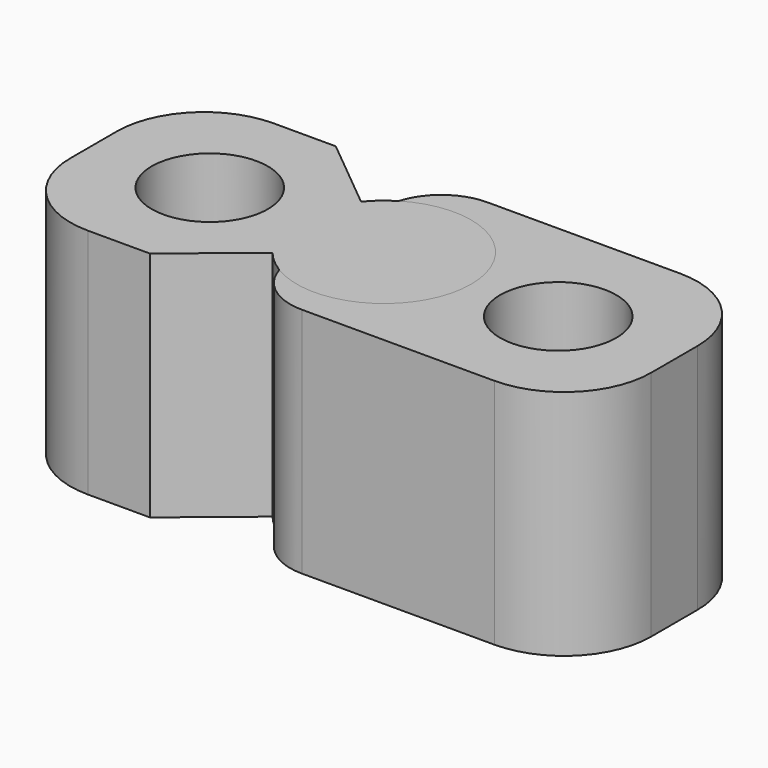
from build123d import *

# Parameters (mm, degrees)
F1_DEPTH    = 4
F2_DEPTH    = 4
F3_R        = 1.5
F3_2_R      = 1.5
F4_T1_DEPTH = 13.1378583471
F5_D        = 2
F5_2_D      = 2


# Not quite as in the source:
# - a fillet or chamfer that OpenCascade refuses, or shapes differently, is made with other operations: its cross-section is extruded or revolved along the edge and cut away or added


with BuildPart() as f1:
    # F0 (on Top) → F1 (new body)
    with BuildSketch(Plane.XY):
        with BuildLine():
            Line((-1.1581599978, 0.9532394345), (-2.4299456272, 2))
            Line((-2.4299456272, 2), (-5, 2))
            Line((-5, 2), (-5, -2))
            Line((-5, -2), (-2.4299456272, -2))
            Line((-2.4299456272, -2), (-1.1581599978, -0.9532394345))
            ThreePointArc((-1.1581599978, -0.9532394345), (-1.5, 0), (-1.1581599978, 0.9532394345))
        make_face()
        with BuildLine():
            ThreePointArc((1.5, 0), (0.7378123545, 1.3059988245), (-0.7741772393, 1.2847760902))
            ThreePointArc((-0.7741772393, 1.2847760902), (-0.9802861511, 1.135358561), (-1.1581599978, 0.9532394345))
            ThreePointArc((-1.1581599978, 0.9532394345), (-1.5, 0), (-1.1581599978, -0.9532394345))
            ThreePointArc((-1.1581599978, -0.9532394345), (-0.9802861511, -1.135358561), (-0.7741772393, -1.2847760902))
            ThreePointArc((-0.7741772393, -1.2847760902), (0.7378123545, -1.3059988245), (1.5, 0))
        make_face()
    extrude(amount=F1_DEPTH)

    # F3
    f3_edges = [f1.edges().sort_by_distance(p)[0] for p in [
        (-5, -2, 2),
        (-5, 2, 2),
    ]]
    fillet(f3_edges, radius=F3_R)

    # F5 (through all)
    with Locations(Plane(origin=(0, 0, 0), x_dir=(1, 0, 0), z_dir=(0, 0, -1))):
        with Locations((3, 0), (-3, 0)):
            Hole(F5_D / 2)


with BuildPart() as f2:
    # F0 (on Top) → F2 (new body)
    with BuildSketch(Plane.XY):
        with BuildLine():
            Line((5, -2), (5, 2))
            Line((5, 2), (-1.6431548453, 2))
            Line((-1.6431548453, 2), (-0.7741772393, 1.2847760902))
            ThreePointArc((-0.7741772393, 1.2847760902), (0.7378123545, 1.3059988245), (1.5, 0))
            ThreePointArc((1.5, 0), (0.7378123545, -1.3059988245), (-0.7741772393, -1.2847760902))
            Line((-0.7741772393, -1.2847760902), (-1.6431548453, -2))
            Line((-1.6431548453, -2), (5, -2))
        make_face()
    extrude(amount=F2_DEPTH)

    # F3#2
    f3_2_edges = [f2.edges().sort_by_distance(p)[0] for p in [
        (5, -2, 2),
        (5, 2, 2),
    ]]
    fillet(f3_2_edges, radius=F3_2_R)

    # F4: fillet of radius 1 on 2 edges, made by hand

    # F4_s2 → F4_t1 (cut)
    with BuildSketch(Plane.XY.offset(-4.5689291735)):
        with BuildLine():
            ThreePointArc((-0.7741772393, 1.2847760902), (-0.4135898271, 1.8014911385), (0.1844168241, 2))
            Line((0.1844168241, 2), (-1.6431548453, 2))
            Line((-1.6431548453, 2), (-0.7741772393, 1.2847760902))
        make_face()
        with BuildLine():
            ThreePointArc((0.1844168241, -2), (-0.4135898271, -1.8014911385), (-0.7741772393, -1.2847760902))
            Line((-0.7741772393, -1.2847760902), (-1.6431548453, -2))
            Line((-1.6431548453, -2), (0.1844168241, -2))
        make_face()
    extrude(amount=F4_T1_DEPTH, mode=Mode.SUBTRACT)

    # F5#2 (through all)
    with Locations(Plane(origin=(0, 0, 0), x_dir=(1, 0, 0), z_dir=(0, 0, -1))):
        with Locations((3, 0), (-3, 0)):
            Hole(F5_2_D / 2)


solid = Compound([f1.part, f2.part])
